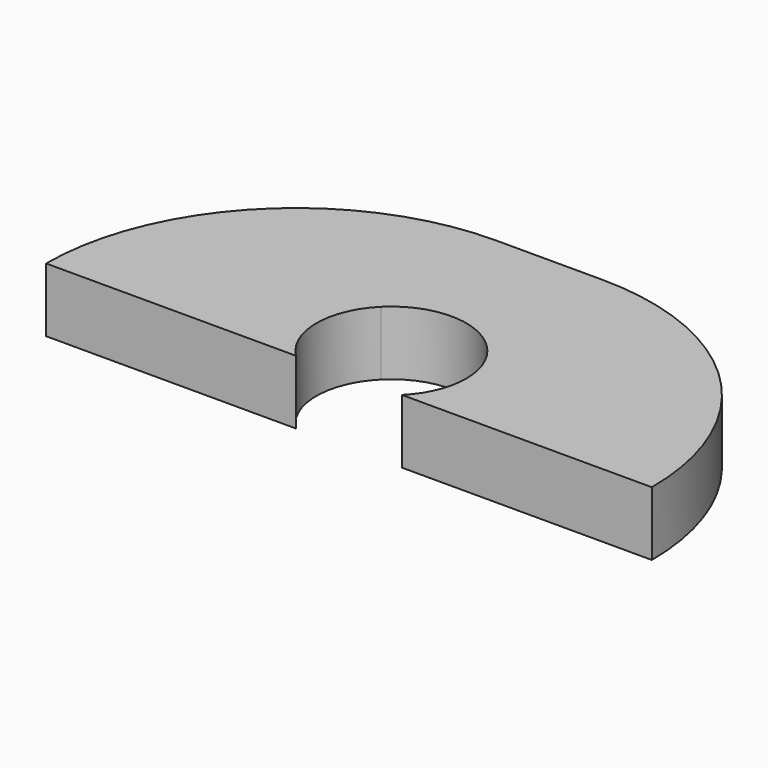
from build123d import *

# Parameters (mm, degrees)
F1_DEPTH = 5


with BuildPart() as f1:
    # F0 (on Top) → F1 (new body)
    with BuildSketch(Plane.XY):
        with BuildLine():
            ThreePointArc((5.8520560333, -5.611971495), (5.4065947922, -7.8514563842), (4.138028505, -9.75))
            Line((4.138028505, -9.75), (9.8424661541, -9.75))
            Line((9.8424661541, -9.75), (12.414085515, -9.75))
            ThreePointArc((12.414085515, -9.75), (9.9900845383, -3.8979439667), (4.138028505, -1.47394299))
            ThreePointArc((4.138028505, -1.47394299), (5.4065947922, -3.3724866058), (5.8520560333, -5.611971495))
        make_face()
        with BuildLine():
            Line((-12.414085515, -9.75), (-4.138028505, -9.75))
            ThreePointArc((-4.138028505, -9.75), (-5.8520560333, -5.611971495), (-4.138028505, -1.47394299))
            ThreePointArc((-4.138028505, -1.47394299), (-9.9900845383, -3.8979439667), (-12.414085515, -9.75))
        make_face()
        with BuildLine():
            ThreePointArc((-4.138028505, -1.47394299), (0, 0.2400845383), (4.138028505, -1.47394299))
            Line((4.138028505, -1.47394299), (4.138028505, 7.9066384221))
            ThreePointArc((4.138028505, 7.9066384221), (2.1083185822, 8.7224970718), (0, 9.305884133))
            ThreePointArc((0, 9.305884133), (-2.1083185822, 8.7224970718), (-4.138028505, 7.9066384221))
            Line((-4.138028505, 7.9066384221), (-4.138028505, -1.47394299))
        make_face()
        with BuildLine():
            Line((4.138028505, 7.9066384221), (4.138028505, -1.47394299))
            ThreePointArc((4.138028505, -1.47394299), (9.9900845383, -3.8979439667), (12.414085515, -9.75))
            Line((12.414085515, -9.75), (15.361971495, -9.75))
            ThreePointArc((15.361971495, -9.75), (12.3184764656, 0.7110441234), (4.138028505, 7.9066384221))
        make_face()
        with BuildLine():
            ThreePointArc((-12.414085515, -9.75), (-9.9900845383, -3.8979439667), (-4.138028505, -1.47394299))
            Line((-4.138028505, -1.47394299), (-4.138028505, 7.9066384221))
            ThreePointArc((-4.138028505, 7.9066384221), (-12.3184764656, 0.7110441234), (-15.361971495, -9.75))
            Line((-15.361971495, -9.75), (-12.414085515, -9.75))
        make_face()
        with BuildLine():
            ThreePointArc((0, 9.305884133), (2.1083185822, 8.7224970718), (4.138028505, 7.9066384221))
            Line((4.138028505, 7.9066384221), (4.138028505, 9.75))
            ThreePointArc((4.138028505, 9.75), (2.057132135, 9.6386531326), (0, 9.305884133))
        make_face()
        with BuildLine():
            Line((4.138028505, 9.75), (4.138028505, 7.9066384221))
            ThreePointArc((4.138028505, 7.9066384221), (12.3184764656, 0.7110441234), (15.361971495, -9.75))
            Line((15.361971495, -9.75), (23.638028505, -9.75))
            ThreePointArc((23.638028505, -9.75), (17.9266107381, 4.0385822331), (4.138028505, 9.75))
        make_face()
        with BuildLine():
            ThreePointArc((-15.361971495, -9.75), (-12.3184764656, 0.7110441234), (-4.138028505, 7.9066384221))
            Line((-4.138028505, 7.9066384221), (-4.138028505, 9.75))
            ThreePointArc((-4.138028505, 9.75), (-17.9266107381, 4.0385822331), (-23.638028505, -9.75))
            Line((-23.638028505, -9.75), (-15.361971495, -9.75))
        make_face()
        with BuildLine():
            Line((-4.138028505, 9.75), (-4.138028505, 7.9066384221))
            ThreePointArc((-4.138028505, 7.9066384221), (-2.1083185822, 8.7224970718), (0, 9.305884133))
            ThreePointArc((0, 9.305884133), (-2.057132135, 9.6386531326), (-4.138028505, 9.75))
        make_face()
        with BuildLine():
            ThreePointArc((0, 9.305884133), (2.057132135, 9.6386531326), (4.138028505, 9.75))
            Line((4.138028505, 9.75), (-4.138028505, 9.75))
            ThreePointArc((-4.138028505, 9.75), (-2.057132135, 9.6386531326), (0, 9.305884133))
        make_face()
    extrude(amount=F1_DEPTH)


solid = f1.part
